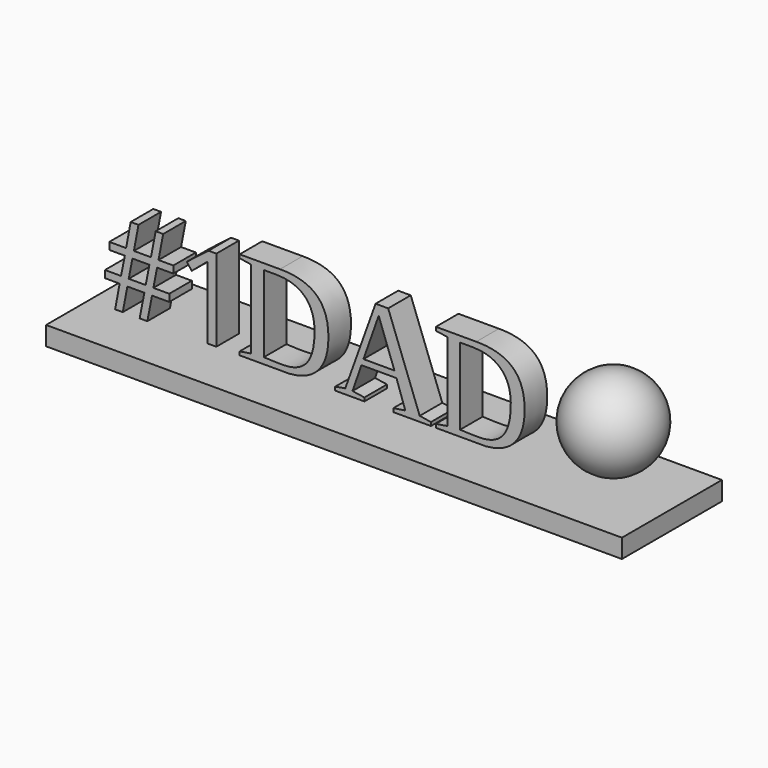
from build123d import *

# Parameters (mm, degrees)
F0_W         = 155.4696410894
F0_H         = 33.7482821196
F1_DEPTH     = 5.08
F2_TEXT_SIZE = 36.6817901118
F3_DEPTH     = 7.62
F4_TEXT_SIZE = 31.0021653099
F5_DEPTH     = 7.62


# Not quite as in the source:
# - Text() gives the source's letters only with a copy of the font that has no kerning and outlines rounded to 1/6400 em; it was checked with that copy


with BuildPart() as f1:
    # F0 (on Top) → F1 (new body)
    with BuildSketch(Plane.XY):
        with Locations((12.4185979366, -5.4035242647)):
            Rectangle(F0_W, F0_H)
    extrude(amount=F1_DEPTH)

    # F2 (on Front) → F3 (join)
    with BuildSketch(Plane.XZ):
        with Locations((-25.8402526379, 5.08)):
            Text('DAD', F2_TEXT_SIZE, font='Tinos', text_align=(TextAlign.LEFT, TextAlign.BOTTOM))
    extrude(amount=F3_DEPTH)


with BuildPart() as f5:
    # F4 (on Front) → F5 (new body)
    with BuildSketch(Plane.XZ):
        with Locations((-61.9236193597, 5.08)):
            Text('#1', F4_TEXT_SIZE, font='Open Sans', text_align=(TextAlign.LEFT, TextAlign.BOTTOM))
    extrude(amount=F5_DEPTH)


with BuildPart() as f7:
    # F6 (on Front) → F7 (revolve)
    with BuildSketch(Plane.XZ):
        with BuildLine():
            Line((70.0251013041, 17.1220325337), (70.0251013041, 29.1640650675))
            ThreePointArc((70.0251013041, 29.1640650675), (57.9830687703, 17.1220325337), (70.0251013041, 5.08))
            Line((70.0251013041, 5.08), (70.0251013041, 17.1220325337))
        make_face()
    revolve(axis=Axis((70.0251013041, 0, 17.1220325337), (0, 0, -1)))


solid = Compound([f1.part, f5.part, f7.part])
